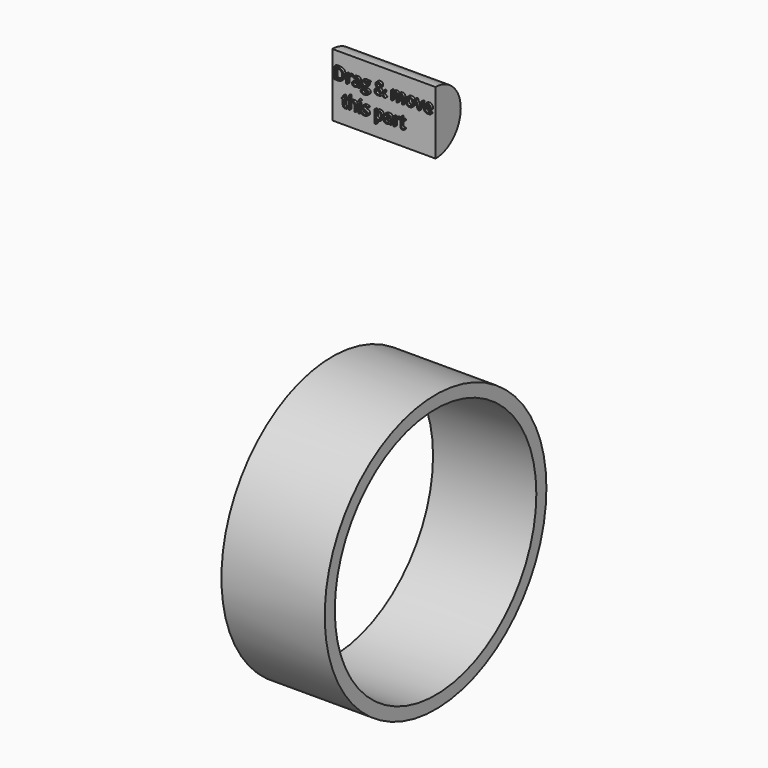
from build123d import *

# Parameters (mm, degrees)
F0_R         = 11
F0_R_2       = 10
F1_DEPTH     = 8.2
F2_TEXT_SIZE = 1.2924941097
F3_DEPTH     = 0.2


# Not quite as in the source:
# - Text() gives the source's letters only with a copy of the font that has no kerning and outlines rounded to 1/6400 em; it was checked with that copy


with BuildPart() as f1:
    # F0 (on Right) → F1 (new body)
    with BuildSketch(Plane.YZ):
        Circle(F0_R)
        Circle(F0_R_2, mode=Mode.SUBTRACT)
    extrude(amount=-F1_DEPTH)


with BuildPart() as f1b:
    # F0 (on Right) → F1, piece 2 (new body)
    with BuildSketch(Plane.YZ):
        with BuildLine():
            Line((0, 32.5), (0, 27.5))
            ThreePointArc((0, 27.5), (2.5, 30), (0, 32.5))
        make_face()
    extrude(amount=-F1_DEPTH)

    # F2 (on face) → F3 (join)
    with BuildSketch(Plane.XZ):
        with Locations((-8, 30.569404241)):
            Text('Drag & move', F2_TEXT_SIZE, font='Open Sans', text_align=(TextAlign.LEFT, TextAlign.BOTTOM))
        with Locations((-7.3283069674, 28.8116122518)):
            Text('this part', F2_TEXT_SIZE, font='Open Sans', text_align=(TextAlign.LEFT, TextAlign.BOTTOM))
    extrude(amount=F3_DEPTH)


solid = Compound([f1.part, f1b.part])
